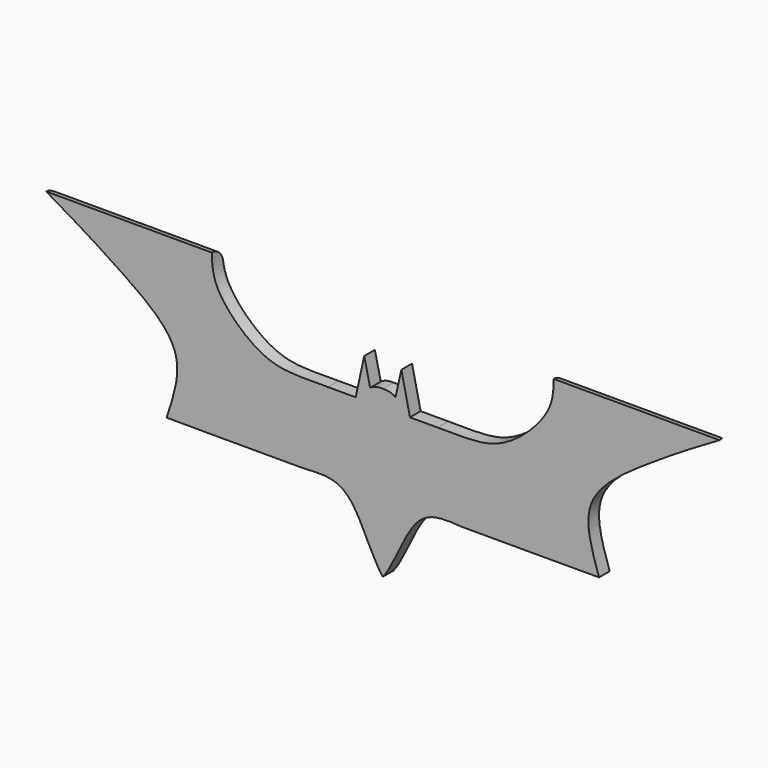
from build123d import *

# Parameters (mm, degrees)
F1_DEPTH = 12.7
F2_R     = 12.69999
F3_R     = 12.69999


# Not quite as in the source:
# - a fillet or chamfer is up to 0.001 mm smaller than in the source, because OpenCascade refuses the exact size


with BuildPart() as f1:
    # F0 (on Front) → F1 (new body)
    with BuildSketch(Plane.XZ):
        with BuildLine():
            add(Edge.make_bspline(
                [(0, 22.1556201577), (4.6081906185, 22.4393960088), (8.8232094422, 21.4276518673), (12.0959098929, 19.0737502837)],
                knots=[0, 0, 0, 0, 12.4823458556, 12.4823458556, 12.4823458556, 12.4823458556], degree=3))
            add(Edge.make_bspline(
                [(0, 22.1556201577), (-4.6081906185, 22.4393960088), (-8.8232094422, 21.4276518673), (-12.0959098929, 19.0737502837)],
                knots=[0, 0, 0, 0, 12.4823458556, 12.4823458556, 12.4823458556, 12.4823458556], degree=3))
            Line((-12.0959098929, 19.0737502837), (-17.7139695734, 43.9015217125))
            Line((-17.7139695734, 43.9015217125), (-25.8638337255, 6.609717384))
            Line((-25.8638337255, 6.609717384), (-52.1656684577, 6.609717384))
            add(Edge.make_bspline(
                [(-52.1656684577, 6.609717384), (-60.3978514517, 6.5219254793), (-78.5756597545, 6.3269402408), (-116.4466347426, 8.1732890136), (-162.2561628931, 52.1737802861), (-162.6985337077, 74.2627820904), (-162.8867536783, 83.3681735719)],
                knots=[0, 0, 0, 0, 0.2084568336, 0.4601327492, 0.7768832352, 1, 1, 1, 1], degree=3))
            Line((-162.8867536783, 83.3681735719), (-320.8426764241, 83.3681735719))
            add(Edge.make_bspline(
                [(-320.8426764241, 83.3681735719), (-310.9533159528, 77.5358259805), (-288.6959219459, 64.6452840474), (-244.3194495003, 36.5716752771), (-184.7380258313, -6.777248073), (-199.2239955574, -48.5914785577), (-206.0440058214, -69.0696899563)],
                knots=[0, 0, 0, 0, 0.2057375573, 0.4598387655, 0.7366005134, 1, 1, 1, 1], degree=3))
            Line((-206.0440058214, -69.0696899563), (-152.1980017424, -69.1764205694))
            Line((-152.1980017424, -69.1764205694), (-100.3352329135, -69.1764205694))
            add(Edge.make_bspline(
                [(-100.3352329135, -69.1764205694), (-93.1837151487, -69.1338341935), (-75.4005733711, -70.292076661), (-27.8541687884, -63.5387172898), (-12.4442655786, -120.211944878), (0, -135.5760842562)],
                knots=[0, 0, 0, 0, 0.2530200956, 0.5731929838, 1, 1, 1, 1], degree=3))
            add(Edge.make_bspline(
                [(100.3352329135, -69.1764205694), (93.1837151487, -69.1338341935), (75.4005733711, -70.292076661), (27.8541687884, -63.5387172898), (12.4442655786, -120.211944878), (0, -135.5760842562)],
                knots=[0, 0, 0, 0, 0.2530200956, 0.5731929838, 1, 1, 1, 1], degree=3))
            Line((100.3352329135, -69.1764205694), (152.1980017424, -69.1764205694))
            Line((152.1980017424, -69.1764205694), (206.0440058214, -69.0696899563))
            add(Edge.make_bspline(
                [(320.8426764241, 83.3681735719), (310.9533159528, 77.5358259805), (288.6959219459, 64.6452840474), (244.3194495003, 36.5716752771), (184.7380258313, -6.777248073), (199.2239955574, -48.5914785577), (206.0440058214, -69.0696899563)],
                knots=[0, 0, 0, 0, 0.2057375573, 0.4598387655, 0.7366005134, 1, 1, 1, 1], degree=3))
            Line((320.8426764241, 83.3681735719), (162.8867536783, 83.3681735719))
            add(Edge.make_bspline(
                [(52.1656684577, 6.609717384), (60.3978514517, 6.5219254793), (78.5756597545, 6.3269402408), (116.4466347426, 8.1732890136), (162.2561628931, 52.1737802861), (162.6985337077, 74.2627820904), (162.8867536783, 83.3681735719)],
                knots=[0, 0, 0, 0, 0.2084568336, 0.4601327492, 0.7768832352, 1, 1, 1, 1], degree=3))
            Line((52.1656684577, 6.609717384), (25.8638337255, 6.609717384))
            Line((25.8638337255, 6.609717384), (17.7139695734, 43.9015217125))
            Line((17.7139695734, 43.9015217125), (12.0959098929, 19.0737502837))
        make_face()
    extrude(amount=F1_DEPTH)

    # F2 (radius 12.7 in the source; OpenCascade refuses exactly that, so slightly less here)
    f2_edges = [f1.edges().sort_by_distance(p)[0] for p in [
        (241.864715, 0, 83.368174),
    ]]
    fillet(f2_edges, radius=F2_R)

    # F3 (radius 12.7 in the source; OpenCascade refuses exactly that, so slightly less here)
    f3_edges = [f1.edges().sort_by_distance(p)[0] for p in [
        (-241.864715, 0, 83.368174),
    ]]
    fillet(f3_edges, radius=F3_R)


solid = f1.part
